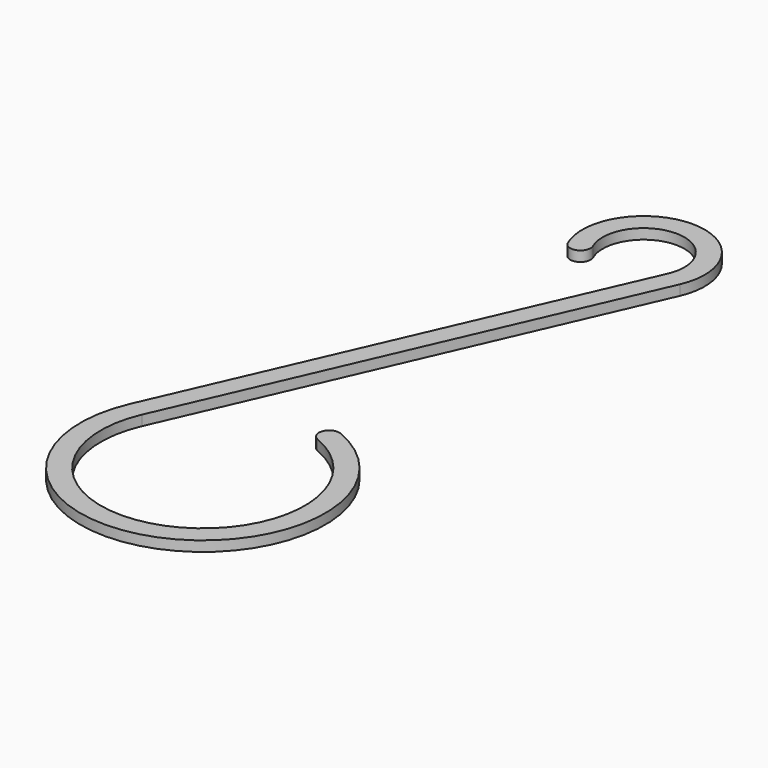
from build123d import *

# Parameters (mm, degrees)
F1_DEPTH = 2


# Not quite as in the source:
# - ends of sketch curves that miss each other by under 0.0002 mm in the source are joined


with BuildPart() as f1:
    # F0 (on Top) → F1 (new body)
    with BuildSketch(Plane.XY):
        with BuildLine():
            Line((-13.3189185158, -36.9739658354), (23.9913511095, 48.1843795013))
            ThreePointArc((23.9913511095, 48.1843795013), (13, 65), (2.0086488905, 48.1843795013))
            ThreePointArc((2.0086488905, 48.1843795013), (4.6431441589, 47.1550910544), (5.6724325972, 49.7895863262))
            ThreePointArc((5.6724325972, 49.7895863262), (12.9999999956, 61), (20.3275674063, 49.7895863342))
            Line((20.3275674063, 49.7895863342), (-16.982702219, -35.3687590025))
            ThreePointArc((-16.982702219, -35.3687590025), (13.8865699132, -67.2941444146), (14.3294887455, -22.8875455965))
            ThreePointArc((14.3294887455, -22.8875455965), (11.7096032974, -23.9521377539), (12.7732628489, -26.5724015487))
            ThreePointArc((12.7732628489, -26.5724015487), (12.4061358524, -63.5781902169), (-13.3189185158, -36.9739658354))
        make_face()
    extrude(amount=F1_DEPTH)


solid = f1.part
